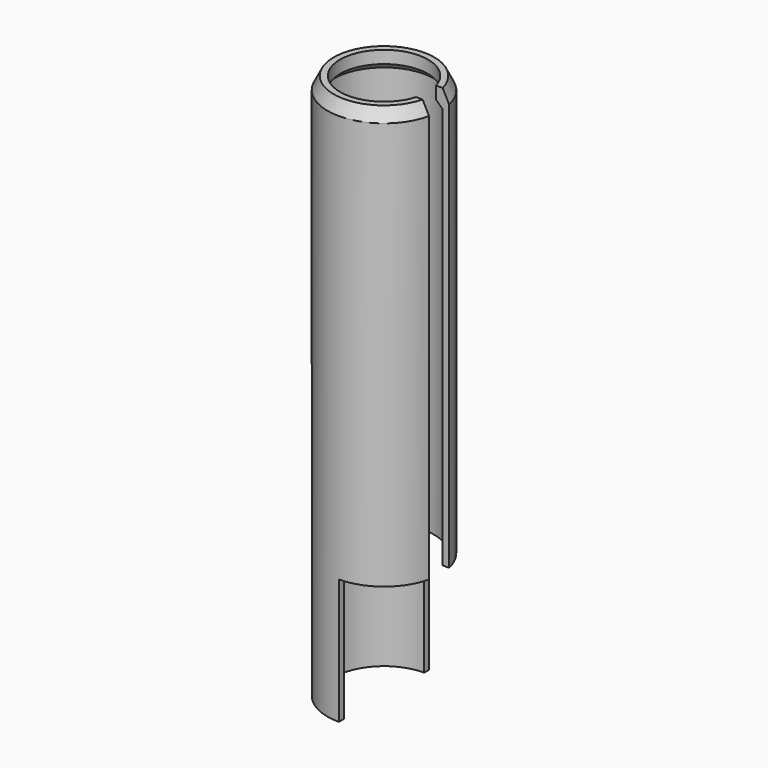
from build123d import *

# Parameters (mm, degrees)
F0_R      = 9
F1_DEPTH  = 40
F3_R      = 9
F4_R      = 8
F6_R      = 8
F8_DEPTH  = 39
F9_R      = 9
F9_R_2    = 8
F10_DEPTH = 45
F12_DEPTH = 20
F13_W     = 4
F13_H     = 4
F14_DEPTH = 100
F7_R      = 7
F15_DEPTH = 25
F16_SIZE2 = 0.99999
F16_SIZE  = 0.99999


# Not quite as in the source:
# - a fillet or chamfer is up to 0.001 mm smaller than in the source, because OpenCascade refuses the exact size


with BuildPart() as f1:
    # F0 (on Top) → F1 (new body)
    with BuildSketch(Plane.XY):
        Circle(F0_R)
    extrude(amount=F1_DEPTH)

    # F3 (on face) → F5 section 0
    with BuildSketch(Plane.XY.offset(40)):
        Circle(F3_R)
    # F4 (on offset) → F5 section 1
    with BuildSketch(Plane.XY.offset(42)):
        Circle(F4_R)
    loft()

    # F6 (on face) → F8 (cut)
    with BuildSketch(Plane(origin=(0, 0, 0), x_dir=(1, 0, 0), z_dir=(0, 0, -1))):
        Circle(F6_R)
    extrude(amount=-F8_DEPTH, mode=Mode.SUBTRACT)

    # F9 (on face) → F10 (join)
    with BuildSketch(Plane(origin=(0, 0, 0), x_dir=(1, 0, 0), z_dir=(0, 0, -1))):
        Circle(F9_R)
        Circle(F9_R_2, mode=Mode.SUBTRACT)
    extrude(amount=F10_DEPTH)

    # F11 (on face) → F12 (cut)
    with BuildSketch(Plane(origin=(0, 0, -45), x_dir=(1, 0, 0), z_dir=(0, 0, -1))):
        with BuildLine():
            ThreePointArc((0, -9), (6.3639610307, -6.3639610307), (9, 0))
            ThreePointArc((9, 0), (6.3639610307, 6.3639610307), (0, 9))
            Line((0, 9), (0, 8))
            ThreePointArc((0, 8), (5.6568542495, 5.6568542495), (8, 0))
            ThreePointArc((8, 0), (5.6568542495, -5.6568542495), (0, -8))
            Line((0, -8), (0, -9))
        make_face()
    extrude(amount=-F12_DEPTH, mode=Mode.SUBTRACT)

    # F13 (on face) → F14 (cut)
    with BuildSketch(Plane(origin=(0, 0, -25), x_dir=(1, 0, 0), z_dir=(0, 0, -1))):
        with Locations((8, 0)):
            Rectangle(F13_W, F13_H)
    extrude(amount=-F14_DEPTH, mode=Mode.SUBTRACT)

    # F7 (on face) → F15 (cut)
    with BuildSketch(Plane.XY.offset(42)):
        Circle(F7_R)
    extrude(amount=-F15_DEPTH, mode=Mode.SUBTRACT)

    # F16 (size 1 and 1 in the source; OpenCascade refuses exactly that, so slightly less here)
    f16_edges = [f1.edges().sort_by_distance(p)[0] for p in [
        (-7, 0, 39),
    ]]
    chamfer(f16_edges, length=F16_SIZE, length2=F16_SIZE2)


solid = f1.part
